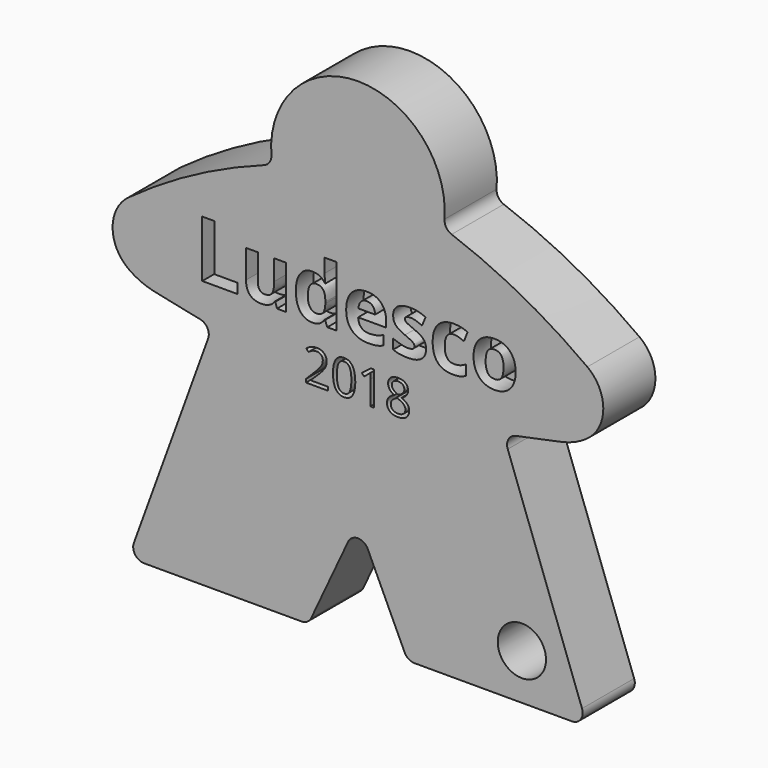
from build123d import *

# Parameters (mm, degrees)
F1_DEPTH       = 3
F3_TEXT_SIZE   = 7.3240511158
F3_TEXT_SIZE_2 = 4.347826087
F4_DEPTH       = 2
F5_TEXT_SIZE   = 5.9133327174
F5_TEXT_SIZE_2 = 4.5030782762
F6_DEPTH       = 2
F7_SCALE       = 0.9
F8_R           = 2
F9_DEPTH       = 25


# Not quite as in the source:
# - Text() gives the source's letters only with a copy of the font that has no kerning and outlines rounded to 1/6400 em; it was checked with that copy


with BuildPart() as f1:
    # F0 (on Front) → F1 (new body, symmetric)
    with BuildSketch(Plane.XZ):
        with BuildLine():
            ThreePointArc((7.9774379507, 19.3995970168), (5.865288734, 25.4404400619), (0, 28))
            ThreePointArc((0, 28), (-5.865288734, 25.4404400619), (-7.9774379507, 19.3995970168))
            ThreePointArc((-7.9774379507, 19.3995970168), (-8.134565282, 18.7820413959), (-8.6328076083, 18.3847775952))
            ThreePointArc((-8.6328076083, 18.3847775952), (-15.1195457534, 15.4884291919), (-21.1303385377, 11.7020092548))
            ThreePointArc((-21.1303385377, 11.7020092548), (-22.6, 8.8), (-21.1303385377, 5.8979907452))
            ThreePointArc((-21.1303385377, 5.8979907452), (-20.0413776914, 5.2628807367), (-18.8437507007, 4.8693200186))
            ThreePointArc((-18.8437507007, 4.8693200186), (-16.6923993699, 4.412393097), (-14.5383700108, 3.9682621703))
            ThreePointArc((-14.5383700108, 3.9682621703), (-13.86498569, 3.4770412758), (-13.7977039581, 2.6462479325))
            Line((-13.7977039581, 2.6462479325), (-20.6418831517, -16.1579798567))
            ThreePointArc((-20.6418831517, -16.1579798567), (-20.5213425752, -17.0735764364), (-19.7021905309, -17.5))
            Line((-19.7021905309, -17.5), (-5.2068853107, -17.5))
            ThreePointArc((-5.2068853107, -17.5), (-4.6695857024, -17.3433914458), (-4.3005775237, -16.9226182617))
            Line((-4.3005775237, -16.9226182617), (-0.906307787, -9.6435833214))
            ThreePointArc((-0.906307787, -9.6435833214), (0, -9.0662015832), (0.906307787, -9.6435833214))
            Line((0.906307787, -9.6435833214), (4.3005775237, -16.9226182617))
            ThreePointArc((4.3005775237, -16.9226182617), (4.6695857024, -17.3433914458), (5.2068853107, -17.5))
            Line((5.2068853107, -17.5), (19.7021905309, -17.5))
            ThreePointArc((19.7021905309, -17.5), (20.5213425752, -17.0735764364), (20.6418831517, -16.1579798567))
            Line((20.6418831517, -16.1579798567), (13.7977039581, 2.6462479325))
            ThreePointArc((13.7977039581, 2.6462479325), (13.86498569, 3.4770412758), (14.5383700108, 3.9682621703))
            ThreePointArc((14.5383700108, 3.9682621703), (16.6923993699, 4.412393097), (18.8437507007, 4.8693200186))
            ThreePointArc((18.8437507007, 4.8693200186), (20.0413776914, 5.2628807367), (21.1303385377, 5.8979907452))
            ThreePointArc((21.1303385377, 5.8979907452), (22.6, 8.8), (21.1303385377, 11.7020092548))
            ThreePointArc((21.1303385377, 11.7020092548), (15.1195457534, 15.4884291919), (8.6328076083, 18.3847775952))
            ThreePointArc((8.6328076083, 18.3847775952), (8.134565282, 18.7820413959), (7.9774379507, 19.3995970168))
        make_face()
    extrude(amount=F1_DEPTH, both=True)

    # F3 (on face) → F4 (cut)
    with BuildSketch(Plane.XZ.offset(3)):
        with Locations((-15, 7.1304347826)):
            Text('Ludesco', F3_TEXT_SIZE, font='Open Sans', font_style=FontStyle.BOLD, text_align=(TextAlign.LEFT, TextAlign.BOTTOM))
        with Locations((-5, 2)):
            Text('2018', F3_TEXT_SIZE_2, font='Open Sans', text_align=(TextAlign.LEFT, TextAlign.BOTTOM))
    extrude(amount=-F4_DEPTH, mode=Mode.SUBTRACT)

    # F5 (on face) → F6 (cut)
    with BuildSketch(Plane(origin=(0, 3, 0), x_dir=(-1, 0, 0), z_dir=(0, 1, 0))):
        with Locations((-10, 7.2422163588)):
            Text('FabLab', F5_TEXT_SIZE, font='Open Sans', text_align=(TextAlign.LEFT, TextAlign.BOTTOM))
        with Locations((-10, 2)):
            Text('ici autour', F5_TEXT_SIZE_2, font='Open Sans', text_align=(TextAlign.LEFT, TextAlign.BOTTOM))
    extrude(amount=-F6_DEPTH, mode=Mode.SUBTRACT)


with BuildPart() as f1_1:
    # F7: moved
    add(f1.part.scale(F7_SCALE))

    # F8 (on face) → F9 (cut)
    with BuildSketch(Plane.XZ.offset(2.7)):
        with Locations((13.5903422583, -11.95)):
            Circle(F8_R)
    extrude(amount=-F9_DEPTH, mode=Mode.SUBTRACT)


solid = f1_1.part
